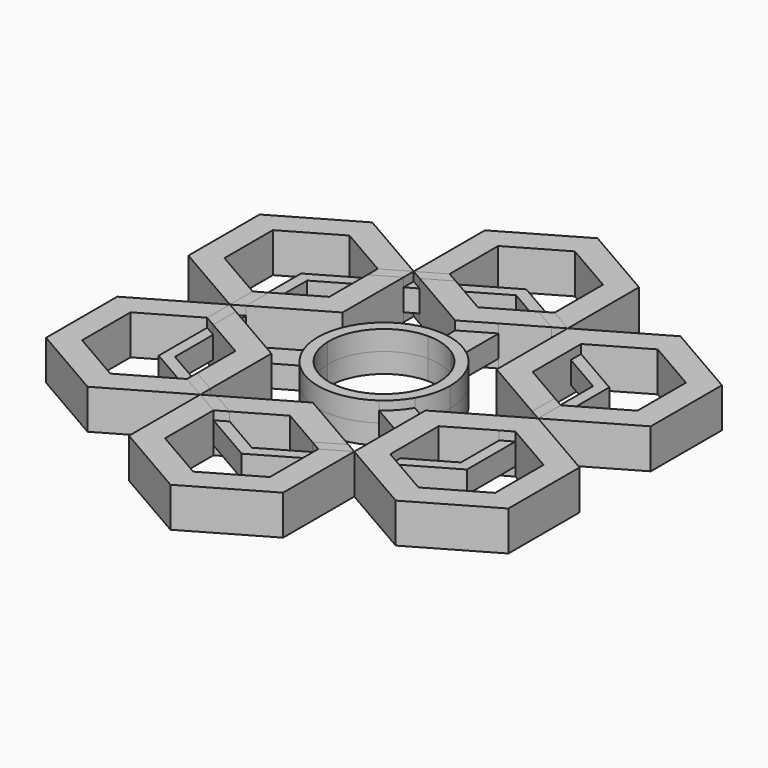
from build123d import *

# Parameters (mm, degrees)
F1_DEPTH      = 4.572
F1_DEPTH_BACK = 4.572
F2_DEPTH      = 2.54
F2_DEPTH_BACK = 2.54
F3_DEPTH      = 4.572
F3_DEPTH_BACK = 4.572
F4_DEPTH      = 2.54
F4_DEPTH_BACK = 2.54


# Not quite as in the source:
# - a feature of the source that left no trace in its solid (it failed there, or was rolled back) is left out


with BuildPart() as f1:
    # F0 (on Top) → F1 (new body, two sides)
    with BuildSketch(Plane.XY) as f1_sk:
        Polygon((-23.4616251091, 27.5155755724), (-17.78, 30.7958633586), (-35.56, 41.0611511448), (-53.34, 30.7958633586), (-53.34, 10.2652877862), (-35.56, 0), (-35.56, 6.5605755724), (-47.6583748909, 13.5455755724), (-47.6583748909, 27.5155755724), (-35.56, 34.5005755724), align=None)
    extrude(amount=F1_DEPTH)
    extrude(f1_sk.sketch, amount=-F1_DEPTH_BACK)


with BuildPart() as f1b:
    # F0 (on Top) → F1, piece 2 (new body, two sides)
    with BuildSketch(Plane.XY) as f1_2_sk:
        Polygon((12.0983748909, 34.0761511448), (17.78, 30.7958633586), (17.78, 51.326438931), (0, 61.5917267171), (-17.78, 51.326438931), (-17.78, 30.7958633586), (-12.0983748909, 34.0761511448), (-12.0983748909, 48.0461511448), (0, 55.0311511448), (12.0983748909, 48.0461511448), align=None)
    extrude(amount=F1_DEPTH)
    extrude(f1_2_sk.sketch, amount=-F1_DEPTH_BACK)


with BuildPart() as f1c:
    # F0 (on Top) → F1, piece 3 (new body, two sides)
    with BuildSketch(Plane.XY) as f1_3_sk:
        Polygon((35.56, 41.0611511448), (17.78, 30.7958633586), (23.4616251091, 27.5155755724), (35.56, 34.5005755724), (47.6583748909, 27.5155755724), (47.6583748909, 13.5455755724), (35.56, 6.5605755724), (35.56, 0), (53.34, 10.2652877862), (53.34, 30.7958633586), align=None)
    extrude(amount=F1_DEPTH)
    extrude(f1_3_sk.sketch, amount=-F1_DEPTH_BACK)



with BuildPart() as f1d:
    # F0 (on Top) → F1, piece 4 (new body, two sides)
    with BuildSketch(Plane.XY) as f1_4_sk:
        Polygon((53.34, -10.2652877862), (35.56, 0), (35.56, -6.5605755724), (47.6583748909, -13.5455755724), (47.6583748909, -27.5155755724), (35.56, -34.5005755724), (23.4616251091, -27.5155755724), (17.78, -30.7958633586), (35.56, -41.0611511448), (53.34, -30.7958633586), align=None)
    extrude(amount=F1_DEPTH)
    extrude(f1_4_sk.sketch, amount=-F1_DEPTH_BACK)



with BuildPart() as f1e:
    # F0 (on Top) → F1, piece 5 (new body, two sides)
    with BuildSketch(Plane.XY) as f1_5_sk:
        Polygon((17.78, -51.326438931), (17.78, -30.7958633586), (12.0983748909, -34.0761511448), (12.0983748909, -48.0461511448), (0, -55.0311511448), (-12.0983748909, -48.0461511448), (-12.0983748909, -34.0761511448), (-17.78, -30.7958633586), (-17.78, -51.326438931), (0, -61.5917267171), align=None)
    extrude(amount=F1_DEPTH)
    extrude(f1_5_sk.sketch, amount=-F1_DEPTH_BACK)


with BuildPart() as f1f:
    # F0 (on Top) → F1, piece 6 (new body, two sides)
    with BuildSketch(Plane.XY) as f1_6_sk:
        Polygon((-35.56, -6.5605755724), (-35.56, 0), (-53.34, -10.2652877862), (-53.34, -30.7958633586), (-35.56, -41.0611511448), (-17.78, -30.7958633586), (-23.4616251091, -27.5155755724), (-35.56, -34.5005755724), (-47.6583748909, -27.5155755724), (-47.6583748909, -13.5455755724), align=None)
    extrude(amount=F1_DEPTH)
    extrude(f1_6_sk.sketch, amount=-F1_DEPTH_BACK)


with BuildPart() as f1g:
    # F0 (on Top) → F1, piece 7 (new body, two sides)
    with BuildSketch(Plane.XY) as f1_7_sk:
        Polygon((-17.78, 10.2652877862), (-17.78, 27.8347122138), (-23.4616251091, 24.5544244276), (-23.4616251091, 13.5455755724), (-32.9955678842, 8.0411511448), (-32.9955678842, 1.4805755724), align=None)
    extrude(amount=F1_DEPTH)
    extrude(f1_7_sk.sketch, amount=-F1_DEPTH_BACK)


with BuildPart() as f1h:
    # F0 (on Top) → F1, piece 8 (new body, two sides)
    with BuildSketch(Plane.XY) as f1_8_sk:
        Polygon((0, 20.5305755724), (6.8690384255, 24.4964167564), (15.2155678842, 29.3152877862), (9.5339427751, 32.5955755724), (0, 27.0911511448), (-9.5339427751, 32.5955755724), (-15.2155678842, 29.3152877862), align=None)
    extrude(amount=F1_DEPTH)
    extrude(f1_8_sk.sketch, amount=-F1_DEPTH_BACK)


with BuildPart() as f1i:
    # F0 (on Top) → F1, piece 9 (new body, two sides)
    with BuildSketch(Plane.XY) as f1_9_sk:
        Polygon((23.4616251091, 24.5544244276), (17.78, 27.8347122138), (17.78, 10.2652877862), (32.9955678842, 1.4805755724), (32.9955678842, 8.0411511448), (23.4616251091, 13.5455755724), align=None)
    extrude(amount=F1_DEPTH)
    extrude(f1_9_sk.sketch, amount=-F1_DEPTH_BACK)


with BuildPart() as f1j:
    # F0 (on Top) → F1, piece 10 (new body, two sides)
    with BuildSketch(Plane.XY) as f1_10_sk:
        Polygon((32.9955678842, -1.4805755724), (17.78, -10.2652877862), (17.78, -17.6346300463), (17.78, -27.8347122138), (23.4616251091, -24.5544244276), (23.4616251091, -13.5455755724), (32.9955678842, -8.0411511448), align=None)
    extrude(amount=F1_DEPTH)
    extrude(f1_10_sk.sketch, amount=-F1_DEPTH_BACK)


with BuildPart() as f1k:
    # F0 (on Top) → F1, piece 11 (new body, two sides)
    with BuildSketch(Plane.XY) as f1_11_sk:
        Polygon((9.5339427751, -32.5955755724), (15.2155678842, -29.3152877862), (0, -20.5305755724), (-15.2155678842, -29.3152877862), (-9.5339427751, -32.5955755724), (0, -27.0911511448), align=None)
    extrude(amount=F1_DEPTH)
    extrude(f1_11_sk.sketch, amount=-F1_DEPTH_BACK)


with BuildPart() as f1l:
    # F0 (on Top) → F1, piece 12 (new body, two sides)
    with BuildSketch(Plane.XY) as f1_12_sk:
        Polygon((-17.78, -10.2652877862), (-23.7722173498, -6.8056794862), (-32.9955678842, -1.4805755724), (-32.9955678842, -8.0411511448), (-23.4616251091, -13.5455755724), (-23.4616251091, -24.5544244276), (-17.78, -27.8347122138), align=None)
    extrude(amount=F1_DEPTH)
    extrude(f1_12_sk.sketch, amount=-F1_DEPTH_BACK)


with BuildPart() as f1m:
    # F0 (on Top) → F1, piece 13 (new body, two sides)
    with BuildSketch(Plane.XY) as f1_13_sk:
        with BuildLine():
            Line((8.7941969643, -12.4466742447), (6.317908423, -11.0169883888))
            ThreePointArc((6.317908423, -11.0169883888), (-3.3048801021, -12.2624535681), (-10.9985226281, -6.35))
            Line((-10.9985226281, -6.35), (-13.1982271537, -7.62))
            ThreePointArc((-13.1982271537, -7.62), (-3.2669659538, -14.8857157522), (8.7941969643, -12.4466742447))
        make_face()
        with BuildLine():
            ThreePointArc((-12.6934020305, -0.4093224793), (-9.1238258282, 8.8343535279), (0, 12.7))
            Line((0, 12.7), (0, 15.24))
            ThreePointArc((0, 15.24), (-11.4005792612, 10.1135746653), (-15.1313135938, -1.8168513767))
            Line((-15.1313135938, -1.8168513767), (-12.6934020305, -0.4093224793))
        make_face()
        with BuildLine():
            ThreePointArc((6.8690384255, 10.6820555657), (11.1473491917, 6.0849491368), (12.7, 0))
            ThreePointArc((12.7, 0), (12.2672579939, -3.2870018728), (10.9985226281, -6.35))
            Line((10.9985226281, -6.35), (13.1982271537, -7.62))
            ThreePointArc((13.1982271537, -7.62), (14.7207095926, -3.9444022474), (15.24, 0))
            ThreePointArc((15.24, 0), (12.9796329995, 7.9866593265), (6.8690384255, 13.6041872638))
            Line((6.8690384255, 13.6041872638), (6.8690384255, 10.6820555657))
        make_face()
        with BuildLine():
            Line((13.1982271537, -7.62), (10.9985226281, -6.35))
            ThreePointArc((10.9985226281, -6.35), (8.9671562517, -8.993336909), (6.317908423, -11.0169883888))
            Line((6.317908423, -11.0169883888), (8.7941969643, -12.4466742447))
            ThreePointArc((8.7941969643, -12.4466742447), (11.2579250181, -10.2721333854), (13.1982271537, -7.62))
        make_face()
        with BuildLine():
            ThreePointArc((0, 12.7), (3.5796574079, 12.1850750035), (6.8690384255, 10.6820555657))
            Line((6.8690384255, 10.6820555657), (6.8690384255, 13.6041872638))
            ThreePointArc((6.8690384255, 13.6041872638), (3.5305655425, 14.8254074801), (0, 15.24))
            Line((0, 15.24), (0, 12.7))
        make_face()
        with BuildLine():
            ThreePointArc((-10.9985226281, -6.35), (-12.2126874953, -3.484288183), (-12.6934020305, -0.4093224793))
            Line((-12.6934020305, -0.4093224793), (-15.1313135938, -1.8168513767))
            ThreePointArc((-15.1313135938, -1.8168513767), (-14.4589022138, -4.8164039254), (-13.1982271537, -7.62))
            Line((-13.1982271537, -7.62), (-10.9985226281, -6.35))
        make_face()
    extrude(amount=F1_DEPTH)
    extrude(f1_13_sk.sketch, amount=-F1_DEPTH_BACK)


with BuildPart() as f2:
    # F0 (on Top) → F2 (new body, two sides)
    with BuildSketch(Plane.XY) as f2_sk:
        with BuildLine():
            ThreePointArc((-13.1982271537, -7.62), (-14.4589022138, -4.8164039254), (-15.1313135938, -1.8168513767))
            Line((-15.1313135938, -1.8168513767), (-23.7722173498, -6.8056794862))
            Line((-23.7722173498, -6.8056794862), (-17.78, -10.2652877862))
            Line((-17.78, -10.2652877862), (-13.1982271537, -7.62))
        make_face()
    extrude(amount=F2_DEPTH)
    extrude(f2_sk.sketch, amount=-F2_DEPTH_BACK)


with BuildPart() as f2b:
    # F0 (on Top) → F2, piece 2 (new body, two sides)
    with BuildSketch(Plane.XY) as f2_2_sk:
        Polygon((-23.4616251091, 24.5544244276), (-23.4616251091, 27.5155755724), (-35.56, 20.5305755724), (-35.56, 6.5605755724), (-32.9955678842, 8.0411511448), (-32.9955678842, 19.05), align=None)
    extrude(amount=F2_DEPTH)
    extrude(f2_2_sk.sketch, amount=-F2_DEPTH_BACK)


with BuildPart() as f2c:
    # F0 (on Top) → F2, piece 3 (new body, two sides)
    with BuildSketch(Plane.XY) as f2_3_sk:
        Polygon((-17.78, 27.8347122138), (-15.2155678842, 29.3152877862), (-17.78, 30.7958633586), align=None)
    extrude(amount=F2_DEPTH)
    extrude(f2_3_sk.sketch, amount=-F2_DEPTH_BACK)


with BuildPart() as f2d:
    # F0 (on Top) → F2, piece 4 (new body, two sides)
    with BuildSketch(Plane.XY) as f2_4_sk:
        Polygon((0, 38.1), (9.5339427751, 32.5955755724), (12.0983748909, 34.0761511448), (0, 41.0611511448), (-12.0983748909, 34.0761511448), (-9.5339427751, 32.5955755724), align=None)
    extrude(amount=F2_DEPTH)
    extrude(f2_4_sk.sketch, amount=-F2_DEPTH_BACK)


with BuildPart() as f1c_1:
    add(f1c.part)

    add(f1i.part)  # F2#5 merges F1i
    # F0 (on Top) → F2, piece 5 (join, two sides)
    with BuildSketch(Plane.XY) as f2_5_sk:
        Polygon((17.78, 30.7958633586), (15.2155678842, 29.3152877862), (17.78, 27.8347122138), align=None)
    extrude(amount=F2_DEPTH)
    extrude(f2_5_sk.sketch, amount=-F2_DEPTH_BACK)

    # F0 (on Top) → F3, piece 11 (join, two sides)
    with BuildSketch(Plane.XY) as f3_11_sk:
        Polygon((23.4616251091, 27.5155755724), (17.78, 30.7958633586), (17.78, 27.8347122138), (23.4616251091, 24.5544244276), align=None)
    extrude(amount=F3_DEPTH)
    extrude(f3_11_sk.sketch, amount=-F3_DEPTH_BACK)


with BuildPart() as f2e:
    # F0 (on Top) → F2, piece 6 (new body, two sides)
    with BuildSketch(Plane.XY) as f2_6_sk:
        Polygon((-15.2155678842, -29.3152877862), (-17.78, -27.8347122138), (-17.78, -30.7958633586), align=None)
    extrude(amount=F2_DEPTH)
    extrude(f2_6_sk.sketch, amount=-F2_DEPTH_BACK)


with BuildPart() as f2f:
    # F0 (on Top) → F2, piece 7 (new body, two sides)
    with BuildSketch(Plane.XY) as f2_7_sk:
        Polygon((-32.9955678842, -19.05), (-32.9955678842, -8.0411511448), (-35.56, -6.5605755724), (-35.56, -20.5305755724), (-23.4616251091, -27.5155755724), (-23.4616251091, -24.5544244276), align=None)
    extrude(amount=F2_DEPTH)
    extrude(f2_7_sk.sketch, amount=-F2_DEPTH_BACK)


with BuildPart() as f2g:
    # F0 (on Top) → F2, piece 8 (new body, two sides)
    with BuildSketch(Plane.XY) as f2_8_sk:
        Polygon((0, -41.0611511448), (12.0983748909, -34.0761511448), (9.5339427751, -32.5955755724), (0, -38.1), (-9.5339427751, -32.5955755724), (-12.0983748909, -34.0761511448), align=None)
    extrude(amount=F2_DEPTH)
    extrude(f2_8_sk.sketch, amount=-F2_DEPTH_BACK)


with BuildPart() as f2h:
    # F0 (on Top) → F2, piece 9 (new body, two sides)
    with BuildSketch(Plane.XY) as f2_9_sk:
        Polygon((35.56, 20.5305755724), (23.4616251091, 27.5155755724), (23.4616251091, 24.5544244276), (32.9955678842, 19.05), (32.9955678842, 8.0411511448), (35.56, 6.5605755724), align=None)
    extrude(amount=F2_DEPTH)
    extrude(f2_9_sk.sketch, amount=-F2_DEPTH_BACK)


with BuildPart() as f1d_1:
    add(f1d.part)

    add(f1j.part)  # F2#10 merges F1j
    # F0 (on Top) → F2, piece 10 (join, two sides)
    with BuildSketch(Plane.XY) as f2_10_sk:
        Polygon((32.9955678842, 1.4805755724), (32.9955678842, -1.4805755724), (35.56, 0), align=None)
        Polygon((17.78, -30.7958633586), (17.78, -27.8347122138), (15.2155678842, -29.3152877862), align=None)
        Polygon((35.56, -6.5605755724), (32.9955678842, -8.0411511448), (32.9955678842, -19.05), (23.4616251091, -24.5544244276), (23.4616251091, -27.5155755724), (35.56, -20.5305755724), align=None)
        with BuildLine():
            Line((17.78, -10.2652877862), (13.1982271537, -7.62))
            ThreePointArc((13.1982271537, -7.62), (11.2579250181, -10.2721333854), (8.7941969643, -12.4466742447))
            Line((8.7941969643, -12.4466742447), (17.78, -17.6346300463))
            Line((17.78, -17.6346300463), (17.78, -10.2652877862))
        make_face()
    extrude(amount=F2_DEPTH)
    extrude(f2_10_sk.sketch, amount=-F2_DEPTH_BACK)

    # F0 (on Top) → F3, piece 10 (join, two sides)
    with BuildSketch(Plane.XY) as f3_10_sk:
        Polygon((23.4616251091, -24.5544244276), (17.78, -27.8347122138), (17.78, -30.7958633586), (23.4616251091, -27.5155755724), align=None)
        Polygon((35.56, 0), (32.9955678842, -1.4805755724), (32.9955678842, -8.0411511448), (35.56, -6.5605755724), align=None)
    extrude(amount=F3_DEPTH)
    extrude(f3_10_sk.sketch, amount=-F3_DEPTH_BACK)


with BuildPart() as f2i:
    # F0 (on Top) → F2, piece 11 (new body, two sides)
    with BuildSketch(Plane.XY) as f2_11_sk:
        with BuildLine():
            ThreePointArc((0, 15.24), (3.5305655425, 14.8254074801), (6.8690384255, 13.6041872638))
            Line((6.8690384255, 13.6041872638), (6.8690384255, 24.4964167564))
            Line((6.8690384255, 24.4964167564), (0, 20.5305755724))
            Line((0, 20.5305755724), (0, 15.24))
        make_face()
    extrude(amount=F2_DEPTH)
    extrude(f2_11_sk.sketch, amount=-F2_DEPTH_BACK)


with BuildPart() as f3:
    # F0 (on Top) → F3 (new body, two sides)
    with BuildSketch(Plane.XY) as f3_sk:
        Polygon((12.0983748909, -34.0761511448), (17.78, -30.7958633586), (15.2155678842, -29.3152877862), (9.5339427751, -32.5955755724), align=None)
    extrude(amount=F3_DEPTH)
    extrude(f3_sk.sketch, amount=-F3_DEPTH_BACK)


with BuildPart() as f3b:
    # F0 (on Top) → F3, piece 2 (new body, two sides)
    with BuildSketch(Plane.XY) as f3_2_sk:
        Polygon((-15.2155678842, -29.3152877862), (-17.78, -30.7958633586), (-12.0983748909, -34.0761511448), (-9.5339427751, -32.5955755724), align=None)
    extrude(amount=F3_DEPTH)
    extrude(f3_2_sk.sketch, amount=-F3_DEPTH_BACK)


with BuildPart() as f3c:
    # F0 (on Top) → F3, piece 3 (new body, two sides)
    with BuildSketch(Plane.XY) as f3_3_sk:
        Polygon((-17.78, -30.7958633586), (-17.78, -27.8347122138), (-23.4616251091, -24.5544244276), (-23.4616251091, -27.5155755724), align=None)
    extrude(amount=F3_DEPTH)
    extrude(f3_3_sk.sketch, amount=-F3_DEPTH_BACK)


with BuildPart() as f3d:
    # F0 (on Top) → F3, piece 4 (new body, two sides)
    with BuildSketch(Plane.XY) as f3_4_sk:
        Polygon((-32.9955678842, -8.0411511448), (-32.9955678842, -1.4805755724), (-35.56, 0), (-35.56, -6.5605755724), align=None)
    extrude(amount=F3_DEPTH)
    extrude(f3_4_sk.sketch, amount=-F3_DEPTH_BACK)


with BuildPart() as f3e:
    # F0 (on Top) → F3, piece 5 (new body, two sides)
    with BuildSketch(Plane.XY) as f3_5_sk:
        Polygon((-35.56, 6.5605755724), (-35.56, 0), (-32.9955678842, 1.4805755724), (-32.9955678842, 8.0411511448), align=None)
    extrude(amount=F3_DEPTH)
    extrude(f3_5_sk.sketch, amount=-F3_DEPTH_BACK)


with BuildPart() as f3f:
    # F0 (on Top) → F3, piece 6 (new body, two sides)
    with BuildSketch(Plane.XY) as f3_6_sk:
        Polygon((-17.78, 27.8347122138), (-17.78, 30.7958633586), (-23.4616251091, 27.5155755724), (-23.4616251091, 24.5544244276), align=None)
    extrude(amount=F3_DEPTH)
    extrude(f3_6_sk.sketch, amount=-F3_DEPTH_BACK)


with BuildPart() as f3g:
    # F0 (on Top) → F3, piece 7 (new body, two sides)
    with BuildSketch(Plane.XY) as f3_7_sk:
        Polygon((-17.78, 30.7958633586), (-15.2155678842, 29.3152877862), (-9.5339427751, 32.5955755724), (-12.0983748909, 34.0761511448), align=None)
    extrude(amount=F3_DEPTH)
    extrude(f3_7_sk.sketch, amount=-F3_DEPTH_BACK)


with BuildPart() as f3h:
    # F0 (on Top) → F3, piece 8 (new body, two sides)
    with BuildSketch(Plane.XY) as f3_8_sk:
        Polygon((9.5339427751, 32.5955755724), (15.2155678842, 29.3152877862), (17.78, 30.7958633586), (12.0983748909, 34.0761511448), align=None)
    extrude(amount=F3_DEPTH)
    extrude(f3_8_sk.sketch, amount=-F3_DEPTH_BACK)


with BuildPart() as f3i:
    # F0 (on Top) → F3, piece 9 (new body, two sides)
    with BuildSketch(Plane.XY) as f3_9_sk:
        Polygon((32.9955678842, 1.4805755724), (35.56, 0), (35.56, 6.5605755724), (32.9955678842, 8.0411511448), align=None)
    extrude(amount=F3_DEPTH)
    extrude(f3_9_sk.sketch, amount=-F3_DEPTH_BACK)


with BuildPart() as f4:
    # F0 (on Top) → F4 (new body, two sides)
    with BuildSketch(Plane.XY) as f4_sk:
        Polygon((-35.56, 0), (-32.9955678842, -1.4805755724), (-32.9955678842, 1.4805755724), align=None)
    extrude(amount=F4_DEPTH)
    extrude(f4_sk.sketch, amount=-F4_DEPTH_BACK)


solid = Compound([f1.part, f1b.part, f1e.part, f1f.part, f1g.part, f1h.part, f1k.part, f1l.part, f1m.part, f2.part, f2b.part, f2c.part, f2d.part, f1c_1.part, f2e.part, f2f.part, f2g.part, f2h.part, f1d_1.part, f2i.part, f3.part, f3b.part, f3c.part, f3d.part, f3e.part, f3f.part, f3g.part, f3h.part, f3i.part, f4.part])
